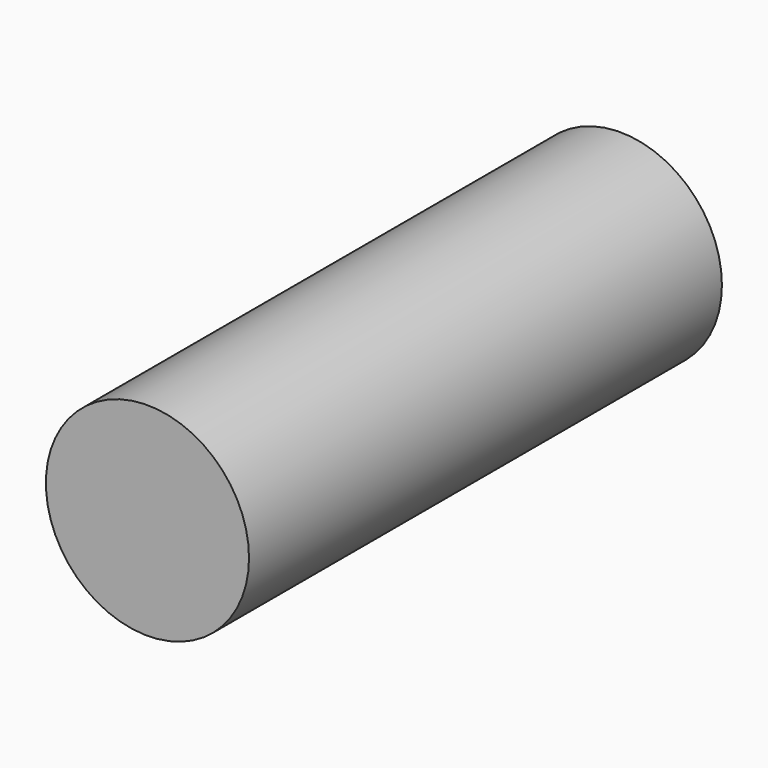
from build123d import *

# Parameters (mm, degrees)
F2_R     = 8.1610092079
F2_R_2   = 4.726237379
F3_DEPTH = 47.498


# Not quite as in the source:
# - the program builds the solid bodies; features that only make, move or delete a surface that nothing else refers to are left out


with BuildPart() as f3:
    # F2 (on Front) → F3 (new body)
    with BuildSketch(Plane.XZ):
        with Locations((12.5965625048, -1.7322285566)):
            Circle(F2_R)
        with Locations((12.5965625048, -1.7322285566)):
            Circle(F2_R_2, mode=Mode.SUBTRACT)
        with Locations((12.5965625048, -1.7322285566)):
            Circle(F2_R_2)
    extrude(amount=F3_DEPTH)


solid = f3.part
